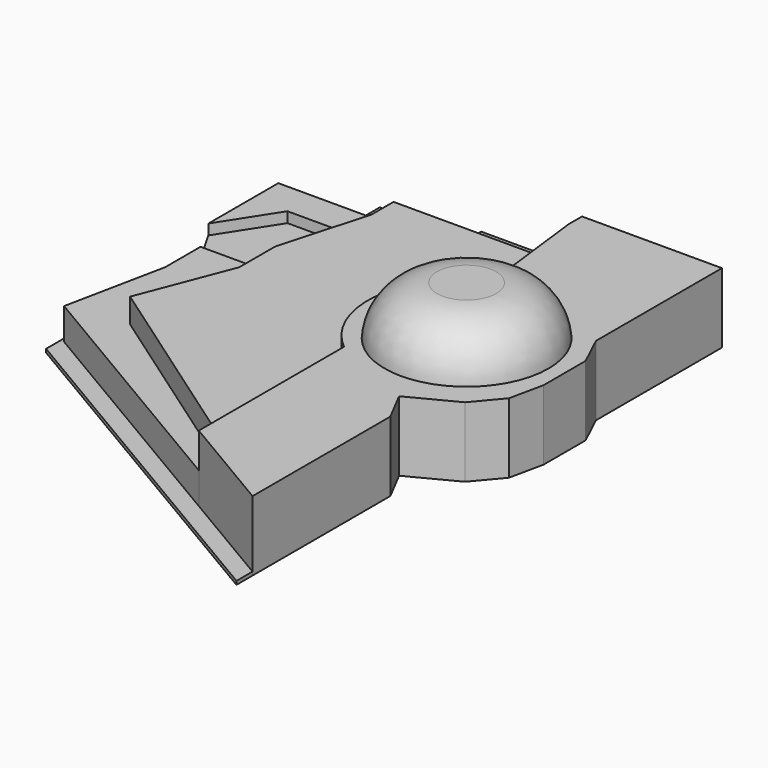
from build123d import *

# Parameters (mm, degrees)
F1_DEPTH = 25.4
F2_DEPTH = 254
F3_DEPTH = 177.8
F4_DEPTH = 431.8
F0_R     = 594.9979970548
F5_DEPTH = 508
F6_DEPTH = 863.6


# Not quite as in the source:
# - a fillet or chamfer that OpenCascade refuses, or shapes differently, is made with other operations: its cross-section is extruded or revolved along the edge and cut away or added


with BuildPart() as f1:
    # F0 (on Top) → F1 (new body)
    with BuildSketch(Plane.XY):
        Polygon((2239.6372437481, -3435.2285861969), (1499.0893602371, -2997.3202280322), (1499.0893602371, -3143.1810455656), (2239.6372437481, -3581.0894037303), align=None)
        Polygon((-357.3869134164, -1899.5296663834), (-208.0992609262, -1169.0624952316), (-383.9827477932, -1233.3211898804), (-383.9827477932, -2029.6635627747), align=None)
        Polygon((1499.0893602371, -2997.3202280322), (-357.3869134164, -1899.5296663834), (-383.9827477932, -2029.6635627747), (1499.0893602371, -3143.1810455656), align=None)
    extrude(amount=F1_DEPTH)

    # F0 (on Top) → F2 (join)
    with BuildSketch(Plane.XY):
        Polygon((333.7312042713, -847.7689027786), (-208.0992609262, -847.7689027786), (-208.0992609262, -1169.0624952316), (-357.3869134164, -1899.5296663834), (1499.0893602371, -2997.3202280322), (1499.0893602371, -2835.1788520813), (75.824059546, -1841.7588472366), (333.7312042713, -1173.1106042862), align=None)
    extrude(amount=F2_DEPTH)


with BuildPart() as f2:
    # F0 (on Top) → F2, piece 2 (new body)
    with BuildSketch(Plane.XY):
        Polygon((283.1003940614, 38.0688405037), (-351.8996059386, 38.0688405037), (-351.8996059386, -596.9311594963), (-96.1140394211, -198.7948268652), (515.2214169502, -198.7948268652), (515.2214169502, 0), (1588.4876312045, 0), (1553.1003940614, 292.0688405037), (918.1003940614, 292.0688405037), (918.1003940614, 165.0688405037), (283.1003940614, 165.0688405037), align=None)
    extrude(amount=F2_DEPTH)


with BuildPart() as f3:
    # F0 (on Top) → F3 (new body)
    with BuildSketch(Plane.XY):
        Polygon((-96.1140394211, -198.7948268652), (-351.8996059386, -596.9311594963), (-208.0992609262, -847.7689027786), (333.7312042713, -847.7689027786), (515.2214169502, -198.7948268652), align=None)
    extrude(amount=F3_DEPTH)


with BuildPart() as f4:
    # F0 (on Top) → F4 (new body)
    with BuildSketch(Plane.XY):
        with BuildLine():
            Line((515.2214169502, -198.7948268652), (333.7312042713, -847.7689027786))
            Line((333.7312042713, -847.7689027786), (333.7312042713, -1173.1106042862))
            Line((333.7312042713, -1173.1106042862), (75.824059546, -1841.7588472366))
            Line((75.824059546, -1841.7588472366), (1499.0893602371, -2835.1788520813))
            Line((1499.0893602371, -2835.1788520813), (1499.0893602371, -1679.3727874756))
            ThreePointArc((1499.0893602371, -1679.3727874756), (1254.6606819019, -1059.0438901467), (1651.9232988358, -523.5667824745))
            Line((1651.9232988358, -523.5667824745), (1588.4876312045, 0))
            Line((1588.4876312045, 0), (515.2214169502, 0))
            Line((515.2214169502, 0), (515.2214169502, -198.7948268652))
        make_face()
    extrude(amount=F4_DEPTH)


with BuildPart() as f5:
    # F0 (on Top) → F5 (new body)
    with BuildSketch(Plane.XY):
        with BuildLine():
            Line((1553.1003940614, 413.4177421996), (1553.1003940614, 292.0688405037))
            Line((1553.1003940614, 292.0688405037), (1588.4876312045, 0))
            Line((1588.4876312045, 0), (1651.9232988358, -523.5667824745))
            ThreePointArc((1651.9232988358, -523.5667824745), (1254.6606819019, -1059.0438901467), (1499.0893602371, -1679.3727874756))
            Line((1499.0893602371, -1679.3727874756), (1499.0893602371, -2835.1788520813))
            Line((1499.0893602371, -2835.1788520813), (1499.0893602371, -2997.3202280322))
            Line((1499.0893602371, -2997.3202280322), (2239.6372437481, -3435.2285861969))
            Line((2239.6372437481, -3435.2285861969), (2239.6372437481, -2184.0894037303))
            Line((2239.6372437481, -2184.0894037303), (2122.4766519932, -1958.7243759651))
            Line((2122.4766519932, -1958.7243759651), (2460.5241936411, -1782.9834883327))
            Line((2460.5241936411, -1782.9834883327), (2624.2396669257, -1588.7845083992))
            Line((2624.2396669257, -1588.7845083992), (2677.2935103517, -1340.3870653815))
            Line((2677.2935103517, -1340.3870653815), (2677.2935103517, -959.3870653815))
            Line((2677.2935103517, -959.3870653815), (2569.1003940614, -729.5822578004))
            Line((2569.1003940614, -729.5822578004), (2569.1003940614, 413.4177421996))
            Line((2569.1003940614, 413.4177421996), (1553.1003940614, 413.4177421996))
        make_face()
        with Locations((1976.6952991486, -1163.5584831238)):
            Circle(F0_R, mode=Mode.SUBTRACT)
    extrude(amount=F5_DEPTH)

    # F0 (on Top) → F6 (join)
    with BuildSketch(Plane.XY):
        with Locations((1976.6952991486, -1163.5584831238)):
            Circle(F0_R)
    extrude(amount=F6_DEPTH)

    # F7: fillet of radius 381 on 1 edges, made by hand

    # F7_s1 → F7_t2 (revolve, cut)
    with BuildSketch(Plane.XZ.offset(1163.5584831238)):
        with BuildLine():
            ThreePointArc((2571.6932962034, 508), (2451.8134551625, 760.8430592126), (2191.5409057072, 863.6))
            Line((2191.5409057072, 863.6), (2571.6932962034, 863.6))
            Line((2571.6932962034, 863.6), (2571.6932962034, 508))
        make_face()
    revolve(axis=Axis((1976.6952991486, -1163.5584831238, 863.6), (0, 0, 1)), mode=Mode.SUBTRACT)


solid = Compound([f1.part, f2.part, f3.part, f4.part, f5.part])
